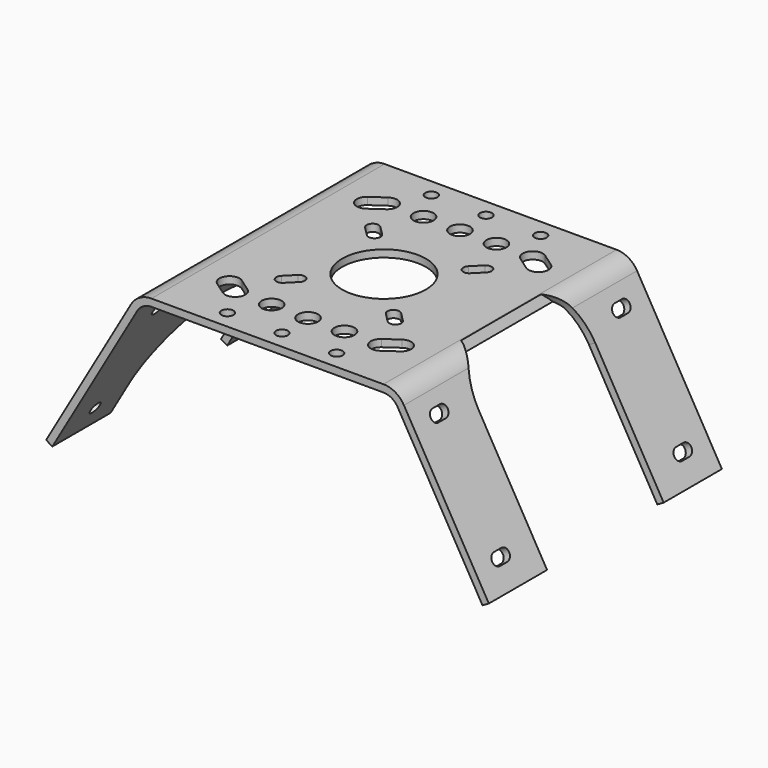
from build123d import *

# Parameters (mm, degrees)
F1_DEPTH = 80
F3_DEPTH = 3
F4_R     = 1.65
F5_DEPTH = 3
F6_R     = 11.5
F6_R_2   = 1.65
F6_R_3   = 2.75
F7_DEPTH = 3


# Not quite as in the source:
# - ends of sketch curves that miss each other by under 0.0002 mm in the source are joined


with BuildPart() as f1:
    # F0 (on Front) → F1 (new body)
    with BuildSketch(Plane.XZ):
        with BuildLine():
            ThreePointArc((-35.747114317, -2.25), (-34.1, -0.602885683), (-31.85, 0))
            Line((-31.85, 0), (31.85, 0))
            ThreePointArc((31.85, 0), (34.1, -0.602885683), (35.747114317, -2.25))
            Line((35.747114317, -2.25), (59.047114317, -42.6067838164))
            Line((59.047114317, -42.6067838164), (60.7791651246, -41.6067838164))
            Line((60.7791651246, -41.6067838164), (37.4791651246, -1.25))
            ThreePointArc((37.4791651246, -1.25), (35.1, 1.1291651246), (31.85, 2))
            Line((31.85, 2), (-31.85, 2))
            ThreePointArc((-31.85, 2), (-35.1, 1.1291651246), (-37.4791651246, -1.25))
            Line((-37.4791651246, -1.25), (-60.7791651246, -41.6067838164))
            Line((-60.7791651246, -41.6067838164), (-59.047114317, -42.6067838164))
            Line((-59.047114317, -42.6067838164), (-35.747114317, -2.25))
        make_face()
    extrude(amount=F1_DEPTH)

    # F2 (on face) → F3 (cut)
    with BuildSketch(Plane(origin=(27.5681079661, 0, 15.9164545553), x_dir=(0, 1, 0), z_dir=(0.8660254038, 0, 0.5))):
        with BuildLine():
            Line((-20, -66.422114317), (-20, -28.8756559143))
            ThreePointArc((-20, -28.8756559143), (-40, -8.8756559143), (-60, -28.8756559143))
            Line((-60, -28.8756559143), (-60, -66.422114317))
            Line((-60, -66.422114317), (-20, -66.422114317))
        make_face()
        with BuildLine():
            Line((-72.5, -60.572114317), (-70, -60.572114317))
            ThreePointArc((-70, -60.572114317), (-68.35, -58.922114317), (-70, -57.272114317))
            Line((-70, -57.272114317), (-72.5, -57.272114317))
            ThreePointArc((-72.5, -57.272114317), (-74.15, -58.922114317), (-72.5, -60.572114317))
        make_face()
        with BuildLine():
            Line((-70.0008798832, -23.522114317), (-72.5008798832, -23.522114317))
            ThreePointArc((-72.5008798832, -23.522114317), (-74.1499997654, -25.1729942001), (-72.499120117, -26.8221140824))
            Line((-72.499120117, -26.8221140824), (-69.9991201168, -26.822114317))
            ThreePointArc((-69.9991201168, -26.822114317), (-68.3500002346, -25.171234434), (-70.0008798832, -23.522114317))
        make_face()
        with BuildLine():
            Line((-9.9999995409, -26.822114317), (-7.4999995409, -26.822114317))
            ThreePointArc((-7.4999995409, -26.822114317), (-5.85, -25.1721140875), (-7.5, -23.522114317))
            Line((-7.5, -23.522114317), (-10, -23.522114317))
            ThreePointArc((-10, -23.522114317), (-11.6499997705, -25.1721145466), (-9.9999995409, -26.822114317))
        make_face()
        with BuildLine():
            Line((-10, -60.572114317), (-7.5, -60.572114317))
            ThreePointArc((-7.5, -60.572114317), (-5.85, -58.922114317), (-7.5, -57.272114317))
            Line((-7.5, -57.272114317), (-10, -57.272114317))
            ThreePointArc((-10, -57.272114317), (-11.65, -58.922114317), (-10, -60.572114317))
        make_face()
    extrude(amount=-F3_DEPTH, mode=Mode.SUBTRACT)

    # F4 (on face) → F5 (cut)
    with BuildSketch(Plane(origin=(-27.5681079661, 0, 15.9164545553), x_dir=(0, -1, 0), z_dir=(-0.8660254038, 0, 0.5))):
        with BuildLine():
            Line((20, -56.422114317), (60, -56.422114317))
            ThreePointArc((60, -56.422114317), (40, -36.422114317), (20, -56.422114317))
        make_face()
        with BuildLine():
            Line((60, -66.422114317), (60, -56.422114317))
            ThreePointArc((60, -56.422114317), (59.3185165258, -61.5984952191), (57.3205080757, -66.422114317))
            Line((57.3205080757, -66.422114317), (60, -66.422114317))
        make_face()
        with BuildLine():
            ThreePointArc((57.3205080757, -66.422114317), (59.3185165258, -61.5984952191), (60, -56.422114317))
            Line((60, -56.422114317), (20, -56.422114317))
            ThreePointArc((20, -56.422114317), (20.6814834742, -61.5984952191), (22.6794919243, -66.422114317))
            Line((22.6794919243, -66.422114317), (57.3205080757, -66.422114317))
        make_face()
        with BuildLine():
            ThreePointArc((22.6794919243, -66.422114317), (20.6814834742, -61.5984952191), (20, -56.422114317))
            Line((20, -56.422114317), (20, -66.422114317))
            Line((20, -66.422114317), (22.6794919243, -66.422114317))
        make_face()
        with BuildLine():
            ThreePointArc((22.6794919243, -66.422114317), (40, -76.422114317), (57.3205080757, -66.422114317))
            Line((57.3205080757, -66.422114317), (22.6794919243, -66.422114317))
        make_face()
        with Locations((70, -58.922114317)):
            Circle(F4_R)
        with Locations((69.7541560233, -25.172114317)):
            Circle(F4_R)
        with Locations((10, -58.922114317)):
            Circle(F4_R)
        with Locations((10, -25.172114317)):
            Circle(F4_R)
    extrude(amount=-F5_DEPTH, mode=Mode.SUBTRACT)

    # F6 (on face) → F7 (cut)
    with BuildSketch(Plane.XY.offset(2)):
        with Locations((0, -40)):
            Circle(F6_R)
        with Locations((-15, -5)):
            Circle(F6_R_2)
        with Locations((0, -5)):
            Circle(F6_R_2)
        with Locations((15, -5)):
            Circle(F6_R_2)
        with Locations((-10, -13.93)):
            Circle(F6_R_3)
        with Locations((0, -13.93)):
            Circle(F6_R_3)
        with Locations((10, -13.93)):
            Circle(F6_R_3)
        with Locations((-10, -66.07)):
            Circle(F6_R_3)
        with Locations((0, -66.07)):
            Circle(F6_R_3)
        with Locations((10, -66.07)):
            Circle(F6_R_3)
        with Locations((0, -75)):
            Circle(F6_R_2)
        with Locations((-15, -75)):
            Circle(F6_R_2)
        with Locations((15, -75)):
            Circle(F6_R_2)
        with BuildLine():
            Line((-18.4225551057, -63.817408691), (-21.9925551057, -61.317408691))
            ThreePointArc((-21.9925551057, -61.317408691), (-25.822591309, -61.9925551057), (-25.1474448943, -65.822591309))
            Line((-25.1474448943, -65.822591309), (-21.5774448943, -68.322591309))
            ThreePointArc((-21.5774448943, -68.322591309), (-17.747408691, -67.6474448943), (-18.4225551057, -63.817408691))
        make_face()
        with BuildLine():
            Line((-21.5774448943, -11.677408691), (-25.1474448943, -14.177408691))
            ThreePointArc((-25.1474448943, -14.177408691), (-25.822591309, -18.0074448943), (-21.9925551057, -18.682591309))
            Line((-21.9925551057, -18.682591309), (-18.4225551057, -16.182591309))
            ThreePointArc((-18.4225551057, -16.182591309), (-17.747408691, -12.3525551057), (-21.5774448943, -11.677408691))
        make_face()
        with BuildLine():
            Line((25.1474448943, -14.177408691), (21.5774448943, -11.677408691))
            ThreePointArc((21.5774448943, -11.677408691), (17.747408691, -12.3525551057), (18.4225551057, -16.182591309))
            Line((18.4225551057, -16.182591309), (21.9925551057, -18.682591309))
            ThreePointArc((21.9925551057, -18.682591309), (25.822591309, -18.0074448943), (25.1474448943, -14.177408691))
        make_face()
        with BuildLine():
            Line((21.9925551057, -61.317408691), (18.4225551057, -63.817408691))
            ThreePointArc((18.4225551057, -63.817408691), (17.747408691, -67.6474448943), (21.5774448943, -68.322591309))
            Line((21.5774448943, -68.322591309), (25.1474448943, -65.822591309))
            ThreePointArc((25.1474448943, -65.822591309), (25.822591309, -61.9925551057), (21.9925551057, -61.317408691))
        make_face()
        with BuildLine():
            Line((-11.833273811, -25.833273811), (-14.333273811, -23.333273811))
            ThreePointArc((-14.333273811, -23.333273811), (-16.666726189, -23.333273811), (-16.666726189, -25.666726189))
            Line((-16.666726189, -25.666726189), (-14.166726189, -28.166726189))
            ThreePointArc((-14.166726189, -28.166726189), (-11.833273811, -28.166726189), (-11.833273811, -25.833273811))
        make_face()
        with BuildLine():
            Line((-14.333273811, -56.666726189), (-11.833273811, -54.166726189))
            ThreePointArc((-11.833273811, -54.166726189), (-11.833273811, -51.833273811), (-14.166726189, -51.833273811))
            Line((-14.166726189, -51.833273811), (-16.666726189, -54.333273811))
            ThreePointArc((-16.666726189, -54.333273811), (-16.666726189, -56.666726189), (-14.333273811, -56.666726189))
        make_face()
        with BuildLine():
            Line((16.666726189, -54.333273811), (14.166726189, -51.833273811))
            ThreePointArc((14.166726189, -51.833273811), (11.833273811, -51.833273811), (11.833273811, -54.166726189))
            Line((11.833273811, -54.166726189), (14.333273811, -56.666726189))
            ThreePointArc((14.333273811, -56.666726189), (16.666726189, -56.666726189), (16.666726189, -54.333273811))
        make_face()
        with BuildLine():
            Line((14.333273811, -23.333273811), (11.833273811, -25.833273811))
            ThreePointArc((11.833273811, -25.833273811), (11.833273811, -28.166726189), (14.166726189, -28.166726189))
            Line((14.166726189, -28.166726189), (16.666726189, -25.666726189))
            ThreePointArc((16.666726189, -25.666726189), (16.666726189, -23.333273811), (14.333273811, -23.333273811))
        make_face()
    extrude(amount=-F7_DEPTH, mode=Mode.SUBTRACT)


solid = f1.part
